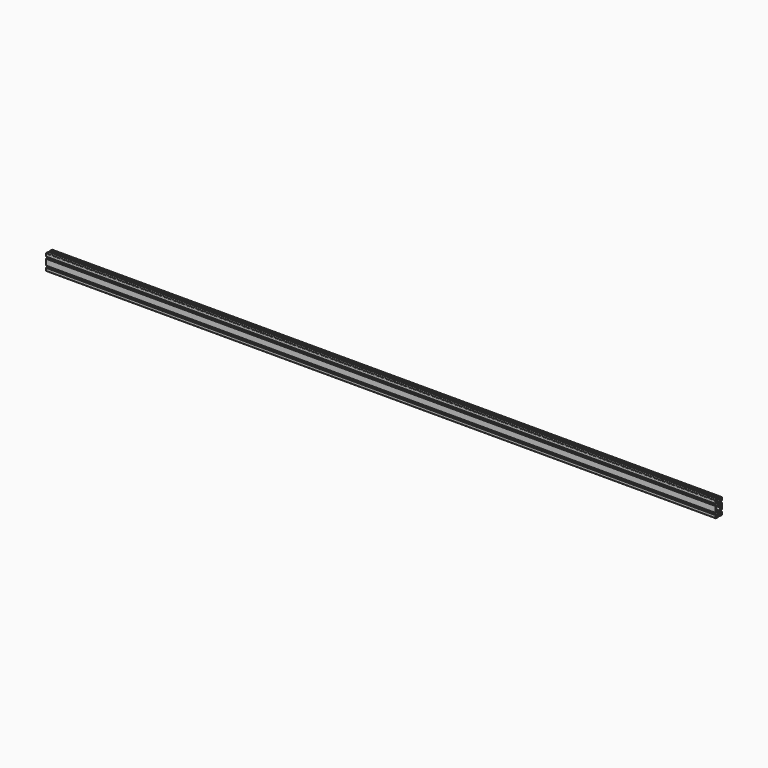
from build123d import *

# Parameters (mm, degrees)
F1_DEPTH = 1676.4


# Not quite as in the source:
# - ends of sketch curves that miss each other by under 0.0002 mm in the source are joined


with BuildPart() as f1:
    # F0 (on Right) → F1 (new body, symmetric)
    with BuildSketch(Plane.YZ):
        with BuildLine():
            Line((-5.6911494, 40.005), (-16.8320974, 40.005))
            ThreePointArc((-16.8320974, 40.005), (-19.0739105776, 39.0764105776), (-20.0025, 36.8345974))
            Line((-20.0025, 36.8345974), (-20.0025, 25.6936494))
            ThreePointArc((-20.0025, 25.6936494), (-19.5425983063, 24.5833484937), (-18.4322974, 24.1234468))
            Line((-18.4322974, 24.1234468), (-17.2521626, 24.1234722))
            ThreePointArc((-17.2521626, 24.1234722), (-16.1418616937, 24.5833484937), (-15.68196, 25.6936494))
            Line((-15.68196, 25.6936494), (-15.68196, 28.7189926))
            ThreePointArc((-15.68196, 28.7189926), (-15.2220583063, 29.8292935063), (-14.1117574, 30.2891952))
            Line((-14.1117574, 30.2891952), (-13.6566148, 30.2891698))
            ThreePointArc((-13.6566148, 30.2891698), (-13.3657390365, 30.2313110133), (-13.1191464712, 30.0665431288))
            Line((-13.1191464712, 30.0665431288), (-9.1109292, 26.0583426))
            ThreePointArc((-9.1109292, 26.0583426), (-8.0562771712, 24.4799853301), (-7.6859384, 22.6181666))
            Line((-7.6859384, 22.6181666), (-7.6859638, 17.3868334))
            ThreePointArc((-7.6859638, 17.3868334), (-8.0562771712, 15.5250146699), (-9.1109127641, 13.9466409641))
            Line((-9.1109127641, 13.9466409641), (-13.1191254, 9.9384358))
            ThreePointArc((-13.1191254, 9.9384358), (-13.36573074, 9.7736670233), (-13.6566148, 9.7158048))
            Line((-13.6566148, 9.7158048), (-14.1117574, 9.7158048))
            ThreePointArc((-14.1117574, 9.7158048), (-15.2220583063, 10.1757064937), (-15.68196, 11.2860074))
            Line((-15.68196, 11.2860074), (-15.68196, 14.3113252))
            ThreePointArc((-15.68196, 14.3113252), (-16.1418616937, 15.4216261063), (-17.2521626, 15.8815278))
            Line((-17.2521626, 15.8815278), (-18.4322974, 15.8815278))
            ThreePointArc((-18.4322974, 15.8815278), (-19.5425983063, 15.4216261063), (-20.0025, 14.3113252))
            Line((-20.0025, 14.3113252), (-20.0025, -14.3113506))
            ThreePointArc((-20.0025, -14.3113506), (-19.5425983063, -15.4216515063), (-18.4322974, -15.8815532))
            Line((-18.4322974, -15.8815532), (-17.2521626, -15.8815278))
            ThreePointArc((-17.2521626, -15.8815278), (-16.1418616937, -15.4216515063), (-15.68196, -14.3113506))
            Line((-15.68196, -14.3113506), (-15.68196, -11.2860074))
            ThreePointArc((-15.68196, -11.2860074), (-15.2220583063, -10.1757064937), (-14.1117574, -9.7158048))
            Line((-14.1117574, -9.7158048), (-13.6566148, -9.7158302))
            ThreePointArc((-13.6566148, -9.7158302), (-13.3657390365, -9.7736889867), (-13.1191464712, -9.9384568712))
            Line((-13.1191464712, -9.9384568712), (-9.1109292, -13.9466574))
            ThreePointArc((-9.1109292, -13.9466574), (-8.0562771712, -15.5250146699), (-7.6859384, -17.3868334))
            Line((-7.6859384, -17.3868334), (-7.6859638, -22.6181666))
            ThreePointArc((-7.6859638, -22.6181666), (-8.0562771712, -24.4799853301), (-9.1109127641, -26.0583590359))
            Line((-9.1109127641, -26.0583590359), (-13.1191254, -30.0665642))
            ThreePointArc((-13.1191254, -30.0665642), (-13.36573074, -30.2313329767), (-13.6566148, -30.2891952))
            Line((-13.6566148, -30.2891952), (-14.1117574, -30.2891952))
            ThreePointArc((-14.1117574, -30.2891952), (-15.2220583063, -29.8292935063), (-15.68196, -28.7189926))
            Line((-15.68196, -28.7189926), (-15.68196, -25.6936748))
            ThreePointArc((-15.68196, -25.6936748), (-16.1418616937, -24.5833738937), (-17.2521626, -24.1234722))
            Line((-17.2521626, -24.1234722), (-18.4322974, -24.1234722))
            ThreePointArc((-18.4322974, -24.1234722), (-19.5425983063, -24.5833738937), (-20.0025, -25.6936748))
            Line((-20.0025, -25.6936748), (-20.0025, -36.8345974))
            ThreePointArc((-20.0025, -36.8345974), (-19.0739105776, -39.0764105776), (-16.8320974, -40.005))
            Line((-16.8320974, -40.005), (-5.6911494, -40.005))
            ThreePointArc((-5.6911494, -40.005), (-4.5808484937, -39.5450983063), (-4.1209468, -38.4347974))
            Line((-4.1209468, -38.4347974), (-4.1209468, -37.2546626))
            ThreePointArc((-4.1209468, -37.2546626), (-4.5808484937, -36.1443616937), (-5.6911494, -35.68446))
            Line((-5.6911494, -35.68446), (-8.7164926, -35.68446))
            ThreePointArc((-8.7164926, -35.68446), (-9.8267935063, -35.2245583063), (-10.2866952, -34.1142574))
            Line((-10.2866952, -34.1142574), (-10.2866698, -33.6591148))
            ThreePointArc((-10.2866698, -33.6591148), (-10.2288144498, -33.368247333), (-10.0640558285, -33.1216591711))
            Line((-10.0640558285, -33.1216591711), (-6.0558426, -29.1134292))
            ThreePointArc((-6.0558426, -29.1134292), (-4.4774770334, -28.0587991346), (-2.6156666, -27.6884638))
            Line((-2.6156666, -27.6884638), (2.6156666, -27.6884638))
            ThreePointArc((2.6156666, -27.6884638), (4.4774770334, -28.0587991346), (6.0558463358, -29.1134254641))
            Line((6.0558463358, -29.1134254641), (10.0640642, -33.1216508))
            ThreePointArc((10.0640642, -33.1216508), (10.2288364133, -33.3682390365), (10.2866952, -33.6591148))
            Line((10.2866952, -33.6591148), (10.2866952, -34.1142574))
            ThreePointArc((10.2866952, -34.1142574), (9.8267935063, -35.2245583063), (8.7164926, -35.68446))
            Line((8.7164926, -35.68446), (5.6911748, -35.68446))
            ThreePointArc((5.6911748, -35.68446), (4.5808738937, -36.1443616937), (4.1209722, -37.2546626))
            Line((4.1209722, -37.2546626), (4.1209722, -38.4347974))
            ThreePointArc((4.1209722, -38.4347974), (4.5808738937, -39.5450983063), (5.6911748, -40.005))
            Line((5.6911748, -40.005), (16.8320974, -40.005))
            ThreePointArc((16.8320974, -40.005), (19.0739105776, -39.0764105776), (20.0025, -36.8345974))
            Line((20.0025, -36.8345974), (20.0025, -25.6936748))
            ThreePointArc((20.0025, -25.6936748), (19.5425983063, -24.5833738937), (18.4322974, -24.1234722))
            Line((18.4322974, -24.1234722), (17.2521626, -24.1234722))
            ThreePointArc((17.2521626, -24.1234722), (16.1418616937, -24.5833738937), (15.68196, -25.6936748))
            Line((15.68196, -25.6936748), (15.68196, -28.7189926))
            ThreePointArc((15.68196, -28.7189926), (15.2220583063, -29.8292935063), (14.1117574, -30.2891952))
            Line((14.1117574, -30.2891952), (13.6566148, -30.2891952))
            ThreePointArc((13.6566148, -30.2891952), (13.3657390365, -30.2313364133), (13.1191464712, -30.0665685288))
            Line((13.1191464712, -30.0665685288), (9.1109292, -26.0583426))
            ThreePointArc((9.1109292, -26.0583426), (8.0562991346, -24.4799770334), (7.6859638, -22.6181666))
            Line((7.6859638, -22.6181666), (7.6859638, -17.3868334))
            ThreePointArc((7.6859638, -17.3868334), (8.0562991346, -15.5250229666), (9.1109254641, -13.9466536642))
            Line((9.1109254641, -13.9466536642), (13.1191508, -9.9384358))
            ThreePointArc((13.1191508, -9.9384358), (13.365747333, -9.7736855502), (13.6566148, -9.7158302))
            Line((13.6566148, -9.7158302), (14.1117574, -9.7158302))
            ThreePointArc((14.1117574, -9.7158302), (15.2220583063, -10.1757064937), (15.68196, -11.2860074))
            Line((15.68196, -11.2860074), (15.68196, -14.3113506))
            ThreePointArc((15.68196, -14.3113506), (16.1418616937, -15.4216515063), (17.2521626, -15.8815532))
            Line((17.2521626, -15.8815532), (18.4322974, -15.8815278))
            ThreePointArc((18.4322974, -15.8815278), (19.5425983063, -15.4216515063), (20.0025, -14.3113506))
            Line((20.0025, -14.3113506), (20.0025, 14.3113252))
            ThreePointArc((20.0025, 14.3113252), (19.5425983063, 15.4216261063), (18.4322974, 15.8815278))
            Line((18.4322974, 15.8815278), (17.2521626, 15.8815278))
            ThreePointArc((17.2521626, 15.8815278), (16.1418616937, 15.4216261063), (15.68196, 14.3113252))
            Line((15.68196, 14.3113252), (15.68196, 11.2860074))
            ThreePointArc((15.68196, 11.2860074), (15.2220583063, 10.1757064937), (14.1117574, 9.7158048))
            Line((14.1117574, 9.7158048), (13.6566148, 9.7158048))
            ThreePointArc((13.6566148, 9.7158048), (13.3657390365, 9.7736635867), (13.1191464712, 9.9384314712))
            Line((13.1191464712, 9.9384314712), (9.1109292, 13.9466574))
            ThreePointArc((9.1109292, 13.9466574), (8.0562991346, 15.5250229666), (7.6859638, 17.3868334))
            Line((7.6859638, 17.3868334), (7.6859638, 22.6181666))
            ThreePointArc((7.6859638, 22.6181666), (8.0562991346, 24.4799770334), (9.1109254641, 26.0583463358))
            Line((9.1109254641, 26.0583463358), (13.1191508, 30.0665642))
            ThreePointArc((13.1191508, 30.0665642), (13.365747333, 30.2313144498), (13.6566148, 30.2891698))
            Line((13.6566148, 30.2891698), (14.1117574, 30.2891698))
            ThreePointArc((14.1117574, 30.2891698), (15.2220583063, 29.8292935063), (15.68196, 28.7189926))
            Line((15.68196, 28.7189926), (15.68196, 25.6936494))
            ThreePointArc((15.68196, 25.6936494), (16.1418616937, 24.5833484937), (17.2521626, 24.1234468))
            Line((17.2521626, 24.1234468), (18.4322974, 24.1234722))
            ThreePointArc((18.4322974, 24.1234722), (19.5425983063, 24.5833484937), (20.0025, 25.6936494))
            Line((20.0025, 25.6936494), (20.0025, 36.8345974))
            ThreePointArc((20.0025, 36.8345974), (19.0739105776, 39.0764105776), (16.8320974, 40.005))
            Line((16.8320974, 40.005), (5.6911748, 40.005))
            ThreePointArc((5.6911748, 40.005), (4.5808738937, 39.5450983063), (4.1209722, 38.4347974))
            Line((4.1209722, 38.4347974), (4.1209722, 37.2546626))
            ThreePointArc((4.1209722, 37.2546626), (4.5808738937, 36.1443616937), (5.6911748, 35.68446))
            Line((5.6911748, 35.68446), (8.7164926, 35.68446))
            ThreePointArc((8.7164926, 35.68446), (9.8267935063, 35.2245583063), (10.2866952, 34.1142574))
            Line((10.2866952, 34.1142574), (10.2866952, 33.6591148))
            ThreePointArc((10.2866952, 33.6591148), (10.2288364133, 33.3682390365), (10.0640685288, 33.1216464712))
            Line((10.0640685288, 33.1216464712), (6.0558426, 29.1134292))
            ThreePointArc((6.0558426, 29.1134292), (4.4774853301, 28.0587771712), (2.6156666, 27.6884384))
            Line((2.6156666, 27.6884384), (-2.6156666, 27.6884638))
            ThreePointArc((-2.6156666, 27.6884638), (-4.4774853301, 28.0587771712), (-6.0558590359, 29.1134127641))
            Line((-6.0558590359, 29.1134127641), (-10.0640642, 33.1216508))
            ThreePointArc((-10.0640642, 33.1216508), (-10.2288144498, 33.368247333), (-10.2866698, 33.6591148))
            Line((-10.2866698, 33.6591148), (-10.2866698, 34.1142574))
            ThreePointArc((-10.2866698, 34.1142574), (-9.8267935063, 35.2245583063), (-8.7164926, 35.68446))
            Line((-8.7164926, 35.68446), (-5.6911494, 35.68446))
            ThreePointArc((-5.6911494, 35.68446), (-4.5808484937, 36.1443616937), (-4.1209468, 37.2546626))
            Line((-4.1209468, 37.2546626), (-4.1209468, 38.4347974))
            ThreePointArc((-4.1209468, 38.4347974), (-4.5808484937, 39.5450983063), (-5.6911494, 40.005))
        make_face()
        with BuildLine():
            ThreePointArc((0, -23.402925), (-2.4044635764, -22.4069635764), (-3.400425, -20.0025))
            ThreePointArc((-3.400425, -20.0025), (-2.4044635764, -17.5980364236), (0, -16.602075))
            ThreePointArc((0, -16.602075), (2.4044635764, -17.5980364236), (3.400425, -20.0025))
            ThreePointArc((3.400425, -20.0025), (2.4044635764, -22.4069635764), (0, -23.402925))
        make_face(mode=Mode.SUBTRACT)
        with BuildLine():
            Line((-15.68196, -4.071874), (-15.68196, 4.0718486))
            ThreePointArc((-15.68196, 4.0718486), (-15.3099409752, 4.9699819752), (-14.4118076, 5.342001))
            Line((-14.4118076, 5.342001), (-12.1314972, 5.3420264))
            ThreePointArc((-12.1314972, 5.3420264), (-11.6454392166, 5.4387075579), (-11.2333765249, 5.7140327249))
            Line((-11.2333765249, 5.7140327249), (-6.0558426, 10.8915708))
            ThreePointArc((-6.0558426, 10.8915708), (-4.4774770334, 11.9462008654), (-2.6156666, 12.3165362))
            Line((-2.6156666, 12.3165362), (2.6156666, 12.3165362))
            ThreePointArc((2.6156666, 12.3165362), (4.4774770334, 11.9462008654), (6.0558463358, 10.8915745359))
            Line((6.0558463358, 10.8915745359), (11.2333786, 5.7140348))
            ThreePointArc((11.2333786, 5.7140348), (11.6454563199, 5.4387109945), (12.1315226, 5.3420264))
            Line((12.1315226, 5.3420264), (14.4118076, 5.3420264))
            ThreePointArc((14.4118076, 5.3420264), (15.3099409752, 4.9699819752), (15.68196, 4.0718486))
            Line((15.68196, 4.0718486), (15.68196, -4.071874))
            ThreePointArc((15.68196, -4.071874), (15.3099409752, -4.9700073752), (14.4118076, -5.3420264))
            Line((14.4118076, -5.3420264), (12.1315226, -5.3420264))
            ThreePointArc((12.1315226, -5.3420264), (11.6454563199, -5.4387109945), (11.2333892248, -5.7140454248))
            Line((11.2333892248, -5.7140454248), (6.0558426, -10.8915708))
            ThreePointArc((6.0558426, -10.8915708), (4.4774853301, -11.9462228288), (2.6156666, -12.3165616))
            Line((2.6156666, -12.3165616), (-2.6156666, -12.3165362))
            ThreePointArc((-2.6156666, -12.3165362), (-4.4774853301, -11.9462228288), (-6.0558590359, -10.8915872359))
            Line((-6.0558590359, -10.8915872359), (-11.2333786, -5.7140348))
            ThreePointArc((-11.2333786, -5.7140348), (-11.6454392166, -5.4387075579), (-12.1314972, -5.3420264))
            Line((-12.1314972, -5.3420264), (-14.4118076, -5.3420264))
            ThreePointArc((-14.4118076, -5.3420264), (-15.3099409752, -4.9700073752), (-15.68196, -4.071874))
        make_face(mode=Mode.SUBTRACT)
        with BuildLine():
            ThreePointArc((0, 16.602075), (-2.4044635764, 17.5980364236), (-3.400425, 20.0025))
            ThreePointArc((-3.400425, 20.0025), (-2.4044635764, 22.4069635764), (0, 23.402925))
            ThreePointArc((0, 23.402925), (2.4044635764, 22.4069635764), (3.400425, 20.0025))
            ThreePointArc((3.400425, 20.0025), (2.4044635764, 17.5980364236), (0, 16.602075))
        make_face(mode=Mode.SUBTRACT)
    extrude(amount=F1_DEPTH, both=True)


solid = f1.part
